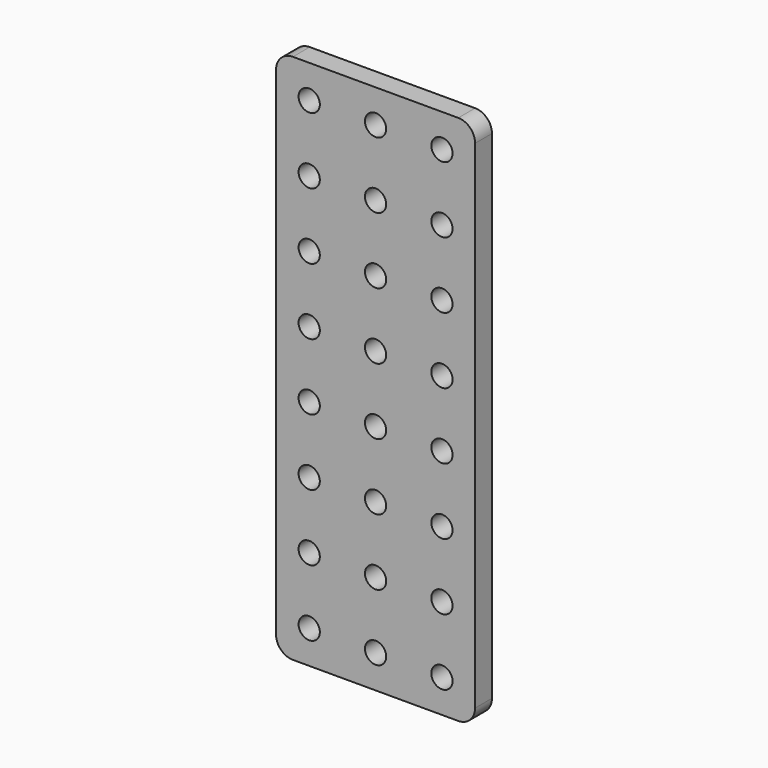
from build123d import *

# Parameters (mm, degrees)
F0_R     = 1.6
F1_DEPTH = 3.175


# Not quite as in the source:
# - a length typed as a fraction of an inch, garbled in the dataset ("3 / 203.2 mm" for 3/8 in), is restored


with BuildPart() as f1:
    # F0 (on Front) → F1 (new body)
    with BuildSketch(Plane.XZ):
        with BuildLine():
            Line((27.46, 0), (2.54, 0))
            ThreePointArc((2.54, 0), (0.7439487758, -0.7439487758), (0, -2.54))
            Line((0, -2.54), (0, -77.46))
            ThreePointArc((0, -77.46), (0.7439487758, -79.2560512242), (2.54, -80))
            Line((2.54, -80), (27.46, -80))
            ThreePointArc((27.46, -80), (29.2560512242, -79.2560512242), (30, -77.46))
            Line((30, -77.46), (30, -2.54))
            ThreePointArc((30, -2.54), (29.2560512242, -0.7439487758), (27.46, 0))
        make_face()
        with Locations((5, -75)):
            Circle(F0_R, mode=Mode.SUBTRACT)
        with Locations((5, -65)):
            Circle(F0_R, mode=Mode.SUBTRACT)
        with Locations((15, -75)):
            Circle(F0_R, mode=Mode.SUBTRACT)
        with Locations((15, -65)):
            Circle(F0_R, mode=Mode.SUBTRACT)
        with Locations((5, -55)):
            Circle(F0_R, mode=Mode.SUBTRACT)
        with Locations((5, -45)):
            Circle(F0_R, mode=Mode.SUBTRACT)
        with Locations((15, -55)):
            Circle(F0_R, mode=Mode.SUBTRACT)
        with Locations((15, -45)):
            Circle(F0_R, mode=Mode.SUBTRACT)
        with Locations((25, -75)):
            Circle(F0_R, mode=Mode.SUBTRACT)
        with Locations((25, -65)):
            Circle(F0_R, mode=Mode.SUBTRACT)
        with Locations((25, -55)):
            Circle(F0_R, mode=Mode.SUBTRACT)
        with Locations((25, -45)):
            Circle(F0_R, mode=Mode.SUBTRACT)
        with Locations((5, -35)):
            Circle(F0_R, mode=Mode.SUBTRACT)
        with Locations((5, -25)):
            Circle(F0_R, mode=Mode.SUBTRACT)
        with Locations((15, -35)):
            Circle(F0_R, mode=Mode.SUBTRACT)
        with Locations((15, -25)):
            Circle(F0_R, mode=Mode.SUBTRACT)
        with Locations((5, -15)):
            Circle(F0_R, mode=Mode.SUBTRACT)
        with Locations((5, -5)):
            Circle(F0_R, mode=Mode.SUBTRACT)
        with Locations((15, -15)):
            Circle(F0_R, mode=Mode.SUBTRACT)
        with Locations((15, -5)):
            Circle(F0_R, mode=Mode.SUBTRACT)
        with Locations((25, -35)):
            Circle(F0_R, mode=Mode.SUBTRACT)
        with Locations((25, -25)):
            Circle(F0_R, mode=Mode.SUBTRACT)
        with Locations((25, -15)):
            Circle(F0_R, mode=Mode.SUBTRACT)
        with Locations((25, -5)):
            Circle(F0_R, mode=Mode.SUBTRACT)
    extrude(amount=F1_DEPTH)


solid = f1.part
